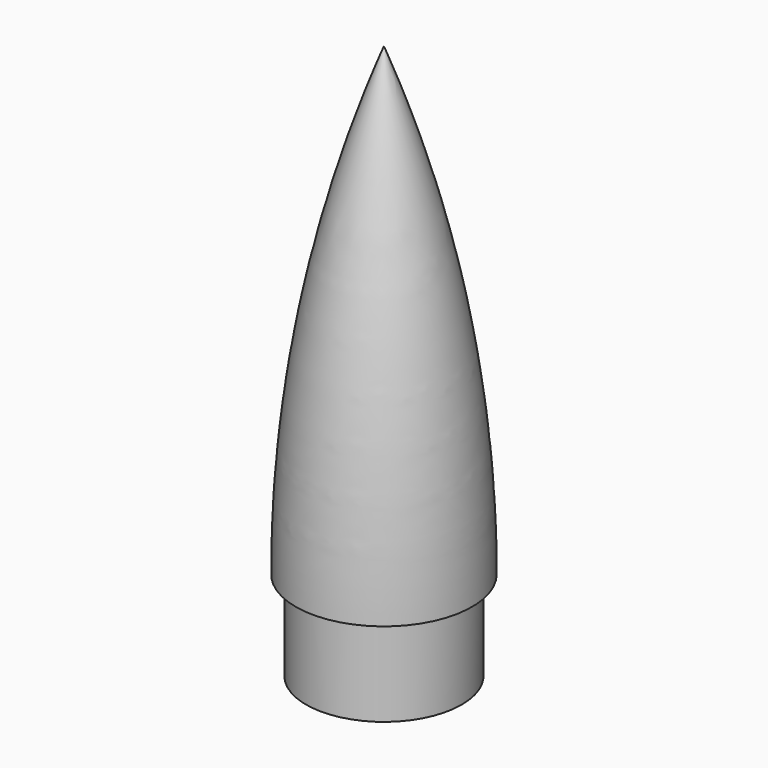
from build123d import *

# Parameters (mm, degrees)
F2_R     = 11.049
F2_R_2   = 8.6868
F3_DEPTH = 12.7
F7_DEPTH = 3.302


# Not quite as in the source:
# - the program builds the solid bodies; features that only make, move or delete a surface that nothing else refers to are left out


with BuildPart() as f1:
    # F0 (on Front) → F1 (revolve)
    with BuildSketch(Plane.XZ):
        with BuildLine():
            Line((0, 59.2769769434), (0, 66.04))
            ThreePointArc((0, 66.04), (-9.3545638677, 33.6071762807), (-12.5095, 0))
            Line((-12.5095, 0), (-10.1473, 0))
            ThreePointArc((-10.1473, 0), (-7.5921575539, 30.0696179426), (0, 59.2769769434))
        make_face()
    revolve(axis=Axis((0, 0, 62.6584884717), (0, 0, 1)))

    # F2 (on Top) → F3 (join)
    with BuildSketch(Plane.XY):
        Circle(F2_R)
        Circle(F2_R_2, mode=Mode.SUBTRACT)
    extrude(amount=-F3_DEPTH)

    # F6 (on Front) → F7 (cut, symmetric)
    with BuildSketch(Plane.XZ):
        with BuildLine():
            ThreePointArc((6.9723, 0), (5.2204583943, 24.7022854782), (0, 48.9101079951))
            ThreePointArc((0, 48.9101079951), (-5.2204583943, 24.7022854782), (-6.9723, 0))
            Line((-6.9723, 0), (0, 0))
            Line((0, 0), (6.9723, 0))
        make_face()
    extrude(amount=F7_DEPTH, both=True, mode=Mode.SUBTRACT)


solid = f1.part
